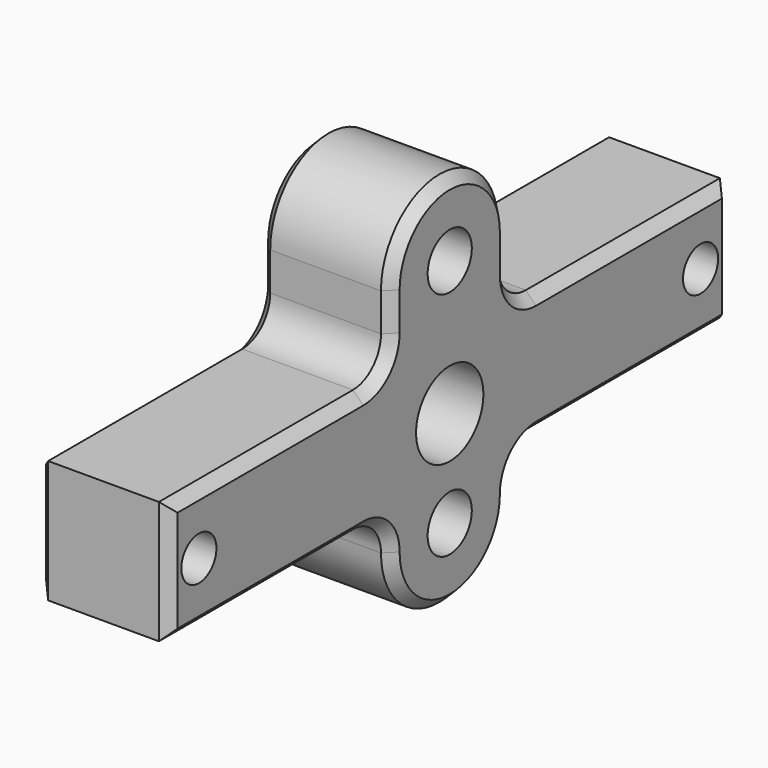
from build123d import *

# Parameters (mm, degrees)
F0_W     = 19.05
F0_H     = 17.78
F1_DEPTH = 50.8
F2_R     = 3.175
F2_R_2   = 6.0964456607
F3_DEPTH = 19.051
F4_R     = 4
F5_DEPTH = 19.05
F6_R     = 5.07999
F7_SIZE  = 1.5


# Not quite as in the source:
# - a fillet or chamfer is up to 0.001 mm smaller than in the source, because OpenCascade refuses the exact size


with BuildPart() as f1:
    # F0 (on Front) → F1 (new body, symmetric)
    with BuildSketch(Plane.XZ):
        Rectangle(F0_W, F0_H)
    extrude(amount=F1_DEPTH, both=True)

    # F2 (on face) → F3 (cut, through all)
    with BuildSketch(Plane.YZ.offset(9.525)):
        with Locations((-45.43298, 0)):
            Circle(F2_R)
        with Locations((45.43298, 0)):
            Circle(F2_R)
        Circle(F2_R_2)
    extrude(amount=-F3_DEPTH, mode=Mode.SUBTRACT)

    # F4 (on face) → F5 (join, through all)
    with BuildSketch(Plane.YZ.offset(9.525)):
        with BuildLine():
            Line((-10.5791, 19.4691), (-10.5791, 8.89))
            Line((-10.5791, 8.89), (10.5791, 8.89))
            Line((10.5791, 8.89), (10.5791, 19.4691))
            ThreePointArc((10.5791, 19.4691), (0, 30.0482), (-10.5791, 19.4691))
        make_face()
        with Locations((0, 19.4691)):
            Circle(F4_R, mode=Mode.SUBTRACT)
        with BuildLine():
            Line((-10.5791, -8.89), (-10.5791, -13.97))
            ThreePointArc((-10.5791, -13.97), (0, -24.5491), (10.5791, -13.97))
            Line((10.5791, -13.97), (10.5791, -8.89))
            Line((10.5791, -8.89), (-10.5791, -8.89))
        make_face()
        with Locations((0, -13.97)):
            Circle(F4_R, mode=Mode.SUBTRACT)
    extrude(amount=-F5_DEPTH)

    # F6 (radius 5.08 in the source; OpenCascade refuses exactly that, so slightly less here)
    f6_edges = [f1.edges().sort_by_distance(p)[0] for p in [
        (0, -10.5791, 8.89),
        (0, 10.5791, 8.89),
        (0, -10.5791, -8.89),
        (0, 10.5791, -8.89),
    ]]
    fillet(f6_edges, radius=F6_R)

    # F7
    f7_edges = [f1.edges().sort_by_distance(p)[0] for p in [
        (9.525, -33.229545, 8.89),
        (9.525, -33.229545, -8.89),
        (-9.525, -33.229545, 8.89),
        (-9.525, -33.229545, -8.89),
        (-9.525, -50.8, 0),
        (-9.525, 50.8, 0),
        (9.525, -50.8, 0),
        (9.525, 50.8, 0),
    ]]
    chamfer(f7_edges, length=F7_SIZE)


solid = f1.part
